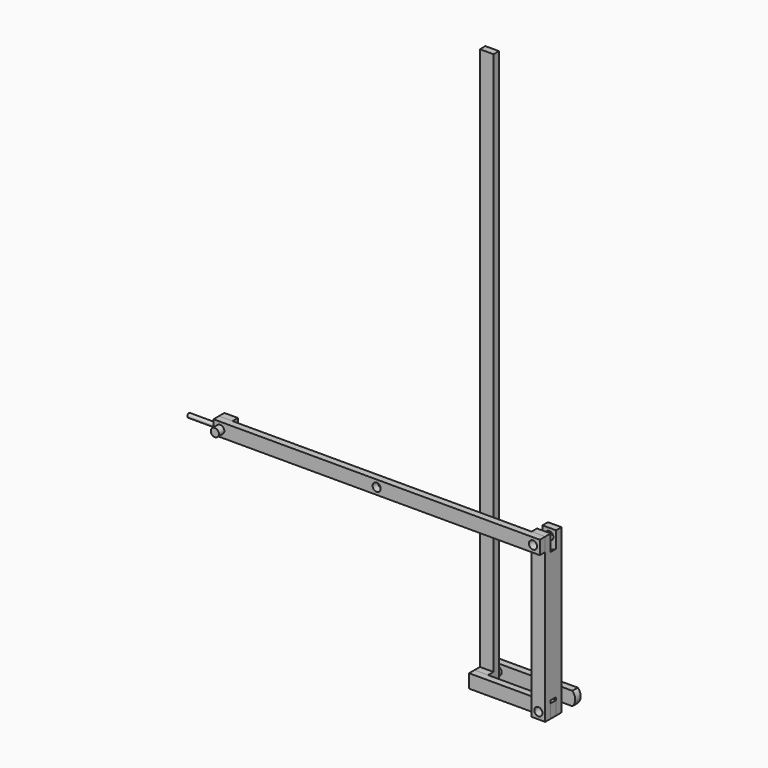
from build123d import *

# Parameters (mm, degrees)
F0_W      = 152.4
F0_H      = 25.4
F0_R      = 7.62
F1_DEPTH  = 6.35
F2_W      = 25.4
F2_H      = 25.4
F2_R      = 7.62
F2_H_2    = 279.4
F3_DEPTH  = 12.7
F5_DEPTH  = 12.7
F6_R      = 7.62
F7_DEPTH  = 12.7
F8_W      = 584.2
F8_H      = 25.4
F8_R      = 7.62
F8_W_2    = 25.4
F9_DEPTH  = 12.7
F10_W     = 25.4
F10_H     = 25.4
F10_R     = 7.62
F11_DEPTH = 25.4
F12_DEPTH = 25.4
F13_W     = 25.4
F13_H     = 12.7
F14_DEPTH = 889
F15_W     = 25.4
F15_H     = 25.4
F15_R     = 7.62
F16_DEPTH = 12.7
F17_DEPTH = 25.4
F18_DEPTH = 127
F19_R     = 3.81
F20_DEPTH = 50.8
F21_DEPTH = 65.024
F22_R     = 7.62
F23_DEPTH = 50.8
F24_R     = 7.62
F25_DEPTH = 12.7


with BuildPart() as f1:
    # F0 (on Front) → F1 (new body, symmetric)
    with BuildSketch(Plane.XZ):
        Rectangle(F0_W, F0_H)
        with Locations((-63.5, 0)):
            Circle(F0_R, mode=Mode.SUBTRACT)
        with Locations((63.5, 0)):
            Circle(F0_R, mode=Mode.SUBTRACT)
    extrude(amount=F1_DEPTH, both=True)

    # F22 (on face) → F23 (join)
    with BuildSketch(Plane.XZ.offset(6.35)):
        with Locations((-63.5, 0)):
            Circle(F22_R)
    extrude(amount=-F23_DEPTH)

    # F24 (on face) → F25 (join)
    with BuildSketch(Plane(origin=(0, 44.45, 0), x_dir=(-1, 0, 0), z_dir=(0, 1, 0))):
        with BuildLine():
            Line((76.2, 12.7), (-76.2, 12.7))
            ThreePointArc((-76.2, 12.7), (-81.4605122421, 0), (-76.2, -12.7))
            Line((-76.2, -12.7), (76.2, -12.7))
            Line((76.2, -12.7), (76.2, 12.7))
        make_face()
        with Locations((63.5, 0)):
            Circle(F24_R, mode=Mode.SUBTRACT)
        with Locations((63.5, 0)):
            Circle(F24_R)
    extrude(amount=F25_DEPTH)


with BuildPart() as f3:
    # F2 (on face) → F3 (new body)
    with BuildSketch(Plane.XZ.offset(6.35)):
        with Locations((63.5, 0)):
            Rectangle(F2_W, F2_H)
        with Locations((63.5, 0)):
            Circle(F2_R, mode=Mode.SUBTRACT)
        with Locations((63.5, 152.4)):
            Rectangle(F2_W, F2_H_2)
        with Locations((63.5, 279.4)):
            Circle(F2_R, mode=Mode.SUBTRACT)
    extrude(amount=F3_DEPTH)

    # F4 (on face) → F5 (join, through all)
    with BuildSketch(Plane.XZ.offset(6.35)):
        with BuildLine():
            Line((50.8, 261.62), (50.8, 17.78))
            ThreePointArc((50.8, 17.78), (63.5, 21.8499061783), (76.2, 17.78))
            Line((76.2, 17.78), (76.2, 261.62))
            ThreePointArc((76.2, 261.62), (63.5, 257.5500938217), (50.8, 261.62))
        make_face()
    extrude(amount=-F5_DEPTH)

    # F6 (on face) → F7 (join)
    with BuildSketch(Plane(origin=(0, 6.35, 0), x_dir=(-1, 0, 0), z_dir=(0, 1, 0))):
        with BuildLine():
            Line((-76.2, -12.7), (-50.8, -12.7))
            Line((-50.8, -12.7), (-50.8, 17.78))
            ThreePointArc((-50.8, 17.78), (-63.5, 21.8499061783), (-76.2, 17.78))
            Line((-76.2, 17.78), (-76.2, -12.7))
        make_face()
        with Locations((-63.5, 0)):
            Circle(F6_R, mode=Mode.SUBTRACT)
        with BuildLine():
            ThreePointArc((-76.2, 17.78), (-63.5, 21.8499061783), (-50.8, 17.78))
            Line((-50.8, 17.78), (-50.8, 261.62))
            ThreePointArc((-50.8, 261.62), (-63.5, 257.5500938217), (-76.2, 261.62))
            Line((-76.2, 261.62), (-76.2, 17.78))
        make_face()
        with BuildLine():
            ThreePointArc((-76.2, 261.62), (-63.5, 257.5500938217), (-50.8, 261.62))
            Line((-50.8, 261.62), (-50.8, 292.1))
            Line((-50.8, 292.1), (-76.2, 292.1))
            Line((-76.2, 292.1), (-76.2, 261.62))
        make_face()
        with Locations((-63.5, 279.4)):
            Circle(F6_R, mode=Mode.SUBTRACT)
    extrude(amount=F7_DEPTH)


with BuildPart() as f9:
    # F8 (on face) → F9 (new body)
    with BuildSketch(Plane.XZ.offset(19.05)):
        with Locations((-241.3, 279.4)):
            Rectangle(F8_W, F8_H)
        with Locations((-520.7, 279.4)):
            Circle(F8_R, mode=Mode.SUBTRACT)
        with Locations((-228.6, 279.4)):
            Circle(F8_R, mode=Mode.SUBTRACT)
        with Locations((63.5, 279.4)):
            Rectangle(F8_W_2, F8_H)
        with Locations((63.5, 279.4)):
            Circle(F8_R, mode=Mode.SUBTRACT)
    extrude(amount=F9_DEPTH)

    # F19 (on face) → F20 (join)
    with BuildSketch(Plane(origin=(-533.4, 0, 0), x_dir=(0, -1, 0), z_dir=(-1, 0, 0))):
        with Locations((25.4, 279.4)):
            Circle(F19_R)
    extrude(amount=F20_DEPTH)


with BuildPart() as f11:
    # F10 (on face) → F11 (new body)
    with BuildSketch(Plane(origin=(0, 6.35, 0), x_dir=(-1, 0, 0), z_dir=(0, 1, 0))):
        with Locations((63.5, 0)):
            Rectangle(F10_W, F10_H)
        with Locations((63.5, 0)):
            Circle(F10_R, mode=Mode.SUBTRACT)
    extrude(amount=-F11_DEPTH)

    # F21 (cut): a face of the model
    f21_faces = [f11.faces().sort_by_distance(p)[0] for p in [
        (-75.8407897552, -19.05, 0),
    ]]
    extrude(f21_faces, amount=-F21_DEPTH, mode=Mode.SUBTRACT)


with BuildPart() as f12:
    # F10 (on face) → F12 (new body)
    with BuildSketch(Plane(origin=(0, 6.35, 0), x_dir=(-1, 0, 0), z_dir=(0, 1, 0))):
        with Locations((63.5, 0)):
            Rectangle(F10_W, F10_H)
        with Locations((63.5, 0)):
            Circle(F10_R, mode=Mode.SUBTRACT)
    extrude(amount=F12_DEPTH)

    # F13 (on face) → F14 (join)
    with BuildSketch(Plane.XY.offset(12.7)):
        with Locations((-63.5, 25.4)):
            Rectangle(F13_W, F13_H)
    extrude(amount=F14_DEPTH)

    # F18 (add): a face of the model
    f18_faces = [f12.faces().sort_by_distance(p)[0] for p in [
        (-63.5, 25.4, 901.7),
    ]]
    extrude(f18_faces, amount=F18_DEPTH)


with BuildPart() as f16:
    # F15 (on face) → F16 (new body)
    with BuildSketch(Plane(origin=(0, -19.05, 0), x_dir=(-1, 0, 0), z_dir=(0, 1, 0))):
        with Locations((520.7, 279.4)):
            Rectangle(F15_W, F15_H)
        with Locations((520.7, 279.4)):
            Circle(F15_R, mode=Mode.SUBTRACT)
        with Locations((520.7, 279.4)):
            Circle(F15_R)
    extrude(amount=F16_DEPTH)

    # F15 (on face) → F17 (join)
    with BuildSketch(Plane(origin=(0, -19.05, 0), x_dir=(-1, 0, 0), z_dir=(0, 1, 0))):
        with Locations((520.7, 279.4)):
            Circle(F15_R)
    extrude(amount=-F17_DEPTH)


solid = Compound([f1.part, f3.part, f9.part, f12.part, f16.part])
